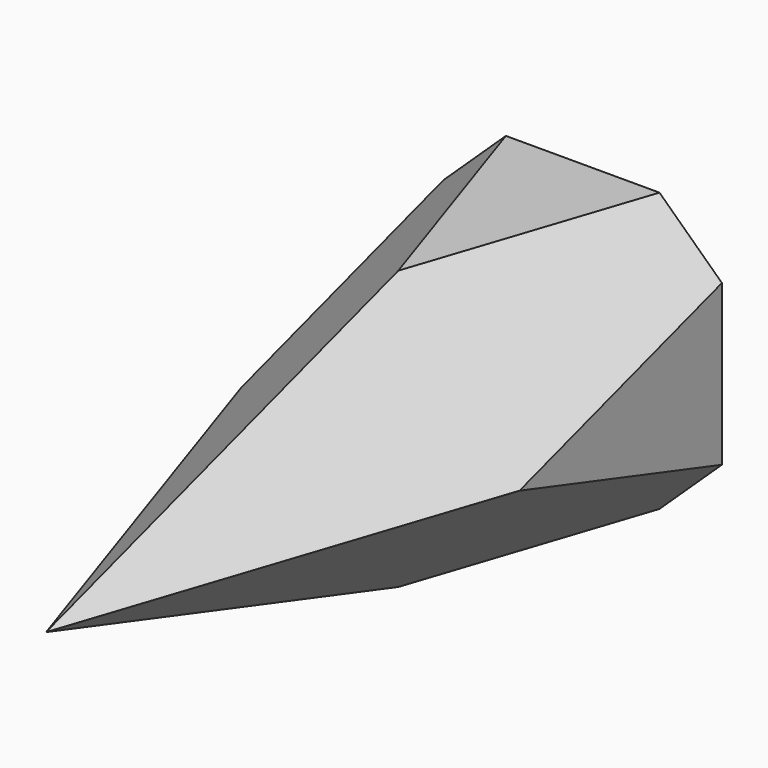
from build123d import *

# Parameters (mm, degrees)
F1_DEPTH = 5
F2_SIZE  = 4.99999


# Not quite as in the source:
# - a fillet or chamfer is up to 0.001 mm smaller than in the source, because OpenCascade refuses the exact size


with BuildPart() as f1:
    # F0 (on Top) → F1 (new body, symmetric)
    with BuildSketch(Plane.XY):
        Polygon((-5, 7.5), (0, -7.5), (5, 7.5), (5, 16.5857542306), (-5, 16.5857542306), align=None)
    extrude(amount=F1_DEPTH, both=True)

    # F2 (size 5 in the source; OpenCascade refuses exactly that, so slightly less here)
    f2_edges = [f1.edges().sort_by_distance(p)[0] for p in [
        (2.5, 0, -5),
        (-2.5, 0, -5),
        (2.5, 0, 5),
        (-2.5, 0, 5),
    ]]
    chamfer(f2_edges, length=F2_SIZE)


solid = f1.part
